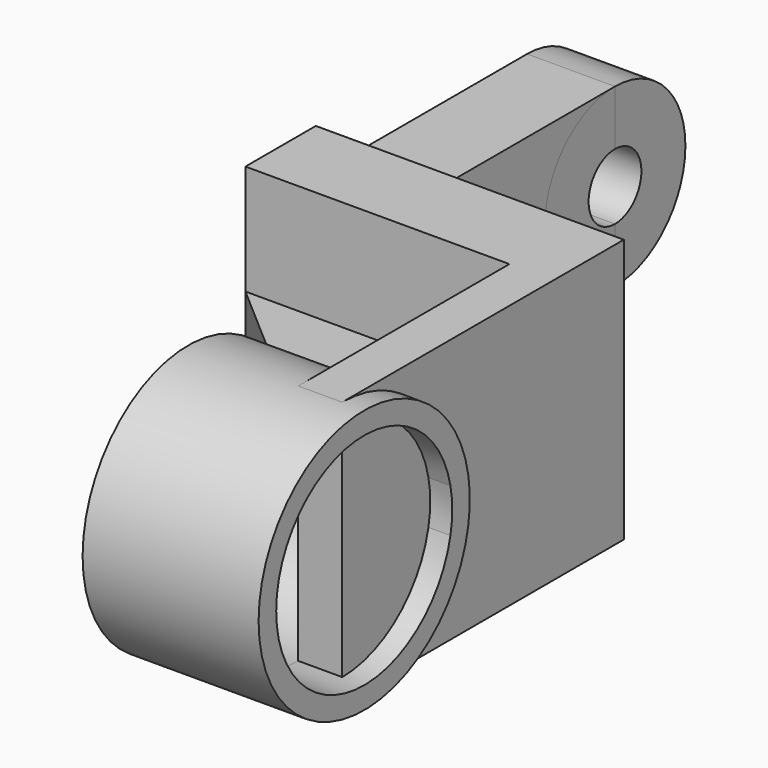
from build123d import *
from build123d import SkipClean  # not in build123d's __all__

# Parameters (mm, degrees)
F0_W      = 70
F0_H      = 60
F8_DEPTH  = 20
F1_W      = 10
F1_H      = 60
F9_DEPTH  = 60
F10_DEPTH = 25
F3_DEPTH  = 40
F4_DEPTH  = 60
F11_DEPTH = 109.889773652
F6_W      = 20
F6_H      = 60
F12_DEPTH = 60
F14_DEPTH = 25
F7_DEPTH  = 20


with BuildPart() as f8:
    # F0 (on Front) → F8 (new body)
    with BuildSketch(Plane.XZ):
        with Locations((-39.945468749, 30)):
            Rectangle(F0_W, F0_H)
    extrude(amount=F8_DEPTH)

    # F1 (on face) → F9 (join)
    with BuildSketch(Plane.XZ.offset(20)):
        with Locations((-9.945468749, 30)):
            Rectangle(F1_W, F1_H)
    extrude(amount=F9_DEPTH)

    # F2 (on face) → F10 (join)
    with BuildSketch(Plane(origin=(-14.945468749, 0, 0), x_dir=(0, -1, 0), z_dir=(-1, 0, 0))):
        with BuildLine():
            Line((55.5051025722, 35), (50.4196010845, 35))
            ThreePointArc((50.4196010845, 35), (50, 30), (50.4196010845, 25))
            Line((50.4196010845, 25), (55.5051025722, 25))
            ThreePointArc((55.5051025722, 25), (55, 30), (55.5051025722, 35))
        make_face()
        with BuildLine():
            Line((55.5051025722, 25), (50.4196010845, 25))
            ThreePointArc((50.4196010845, 25), (60.635083269, 7.0871215252), (80, 0))
            Line((80, 0), (80, 5))
            ThreePointArc((80, 5), (64.1886116992, 10.635083269), (55.5051025722, 25))
        make_face()
        with BuildLine():
            ThreePointArc((80, 60), (60.635083269, 52.9128784748), (50.4196010845, 35))
            Line((50.4196010845, 35), (55.5051025722, 35))
            ThreePointArc((55.5051025722, 35), (64.1886116992, 49.364916731), (80, 55))
            Line((80, 55), (80, 60))
        make_face()
        with BuildLine():
            ThreePointArc((110, 30), (101.2132034356, 51.2132034356), (80, 60))
            Line((80, 60), (80, 55))
            ThreePointArc((80, 55), (97.6776695297, 47.6776695297), (105, 30))
            ThreePointArc((105, 30), (97.6776695297, 12.3223304703), (80, 5))
            Line((80, 5), (80, 0))
            ThreePointArc((80, 0), (101.2132034356, 8.7867965644), (110, 30))
        make_face()
    extrude(amount=F10_DEPTH)

    # F3 (add): a face of the model
    f3_faces = [f8.faces().sort_by_distance(p)[0] for p in [
        (-39.945468749, -80, 4.1514718626),
    ]]
    extrude(f3_faces, amount=-F3_DEPTH)

    # F2 (on face) → F4 (join)
    with BuildSketch(Plane(origin=(-14.945468749, 0, 0), x_dir=(0, -1, 0), z_dir=(-1, 0, 0))):
        with BuildLine():
            Line((50.4196010845, 35), (20, 35))
            Line((20, 35), (20, 25))
            Line((20, 25), (50.4196010845, 25))
            ThreePointArc((50.4196010845, 25), (50, 30), (50.4196010845, 35))
        make_face()
    extrude(amount=F4_DEPTH)

    # F5 (on face) → F11 (cut)
    with BuildSketch(Plane(origin=(0, 0, 25), x_dir=(1, 0, 0), z_dir=(0, 0, -1))):
        Polygon((-74.945468749, 50.4196010845), (-74.945468749, 20), (-39.945468749, 50.4196010845), align=None)
    extrude(amount=-F11_DEPTH, mode=Mode.SUBTRACT)

    # F6 (on face) → F12 (join)
    with BuildSketch(Plane.XZ):
        with Locations((-64.945468749, 30)):
            Rectangle(F6_W, F6_H)
    extrude(amount=-F12_DEPTH)

    # F13 (on face) → F14 (cut)
    with BuildSketch(Plane(origin=(-74.945468749, 0, 0), x_dir=(0, -1, 0), z_dir=(-1, 0, 0))):
        with BuildLine():
            Line((0, 60), (-20, 60))
            ThreePointArc((-20, 60), (-17.0710678119, 52.9289321881), (-10, 50))
            ThreePointArc((-10, 50), (-2.9289321881, 52.9289321881), (0, 60))
        make_face()
        with BuildLine():
            Line((-10, 10), (-60, 10))
            Line((-60, 10), (-60, 0))
            Line((-60, 0), (-20, 0))
            ThreePointArc((-20, 0), (-17.0710678119, 7.0710678119), (-10, 10))
        make_face()
        with BuildLine():
            ThreePointArc((0, 0), (-2.9289321881, 7.0710678119), (-10, 10))
            ThreePointArc((-10, 10), (-17.0710678119, 7.0710678119), (-20, 0))
            Line((-20, 0), (0, 0))
        make_face()
        with BuildLine():
            ThreePointArc((-10, 50), (-17.0710678119, 52.9289321881), (-20, 60))
            Line((-20, 60), (-60, 60))
            Line((-60, 60), (-60, 50))
            Line((-60, 50), (-10, 50))
        make_face()
        with BuildLine():
            ThreePointArc((-52.5, 30), (-54.6966991411, 35.3033008589), (-60, 37.5))
            Line((-60, 37.5), (-60, 22.5))
            ThreePointArc((-60, 22.5), (-54.6966991411, 24.6966991411), (-52.5, 30))
        make_face()
    extrude(amount=-F14_DEPTH, mode=Mode.SUBTRACT)

    # F13 (on face) → F7 (join)
    with BuildSketch(Plane(origin=(-74.945468749, 0, 0), x_dir=(0, -1, 0), z_dir=(-1, 0, 0))):
        with BuildLine():
            Line((-60, 37.5), (-60, 50))
            ThreePointArc((-60, 50), (-80, 30), (-60, 10))
            Line((-60, 10), (-60, 22.5))
            ThreePointArc((-60, 22.5), (-67.5, 30), (-60, 37.5))
        make_face()
        with BuildLine():
            ThreePointArc((-40, 30), (-45.8578643763, 44.1421356237), (-60, 50))
            Line((-60, 50), (-60, 37.5))
            ThreePointArc((-60, 37.5), (-54.6966991411, 35.3033008589), (-52.5, 30))
            ThreePointArc((-52.5, 30), (-54.6966991411, 24.6966991411), (-60, 22.5))
            Line((-60, 22.5), (-60, 10))
            ThreePointArc((-60, 10), (-45.8578643763, 15.8578643763), (-40, 30))
        make_face()
    with SkipClean():  # cleaning this boolean's faces spoils the solid; the shape is the same uncleaned
        extrude(amount=-F7_DEPTH)


solid = f8.part
